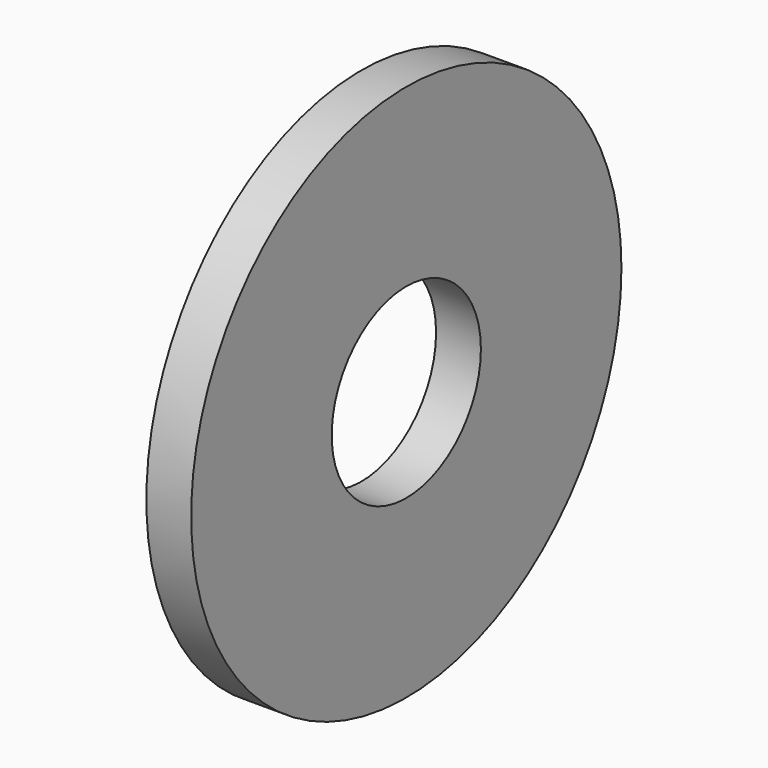
from build123d import *

# Parameters (mm, degrees)
F0_R     = 9.525
F0_R_2   = 3.302
F1_DEPTH = 1.5875


# Not quite as in the source:
# - a length typed as a fraction of an inch, garbled in the dataset ("3 / 203.2 mm" for 3/8 in), is restored


with BuildPart() as f1:
    # F0 (on Right) → F1 (new body)
    with BuildSketch(Plane.YZ):
        Circle(F0_R)
        Circle(F0_R_2, mode=Mode.SUBTRACT)
    extrude(amount=F1_DEPTH)


solid = f1.part
